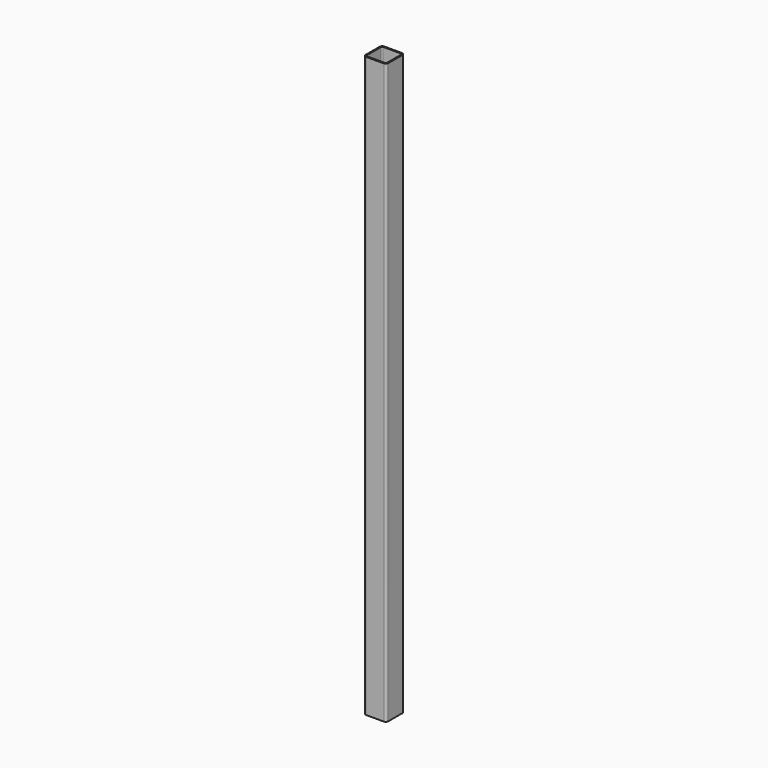
from build123d import *

# Parameters (mm, degrees)
F2_DEPTH = 812.8


# Not quite as in the source:
# - a variable given as a bare number and used for a length is read in inches; the dataset says mm whatever the document's units were


with BuildPart() as f2:
    # F0 (on Top) → F2 (new body)
    with BuildSketch(Plane.XY):
        with BuildLine():
            Line((-12.573, -15.875), (12.573, -15.875))
            ThreePointArc((12.573, -15.875), (14.9078665915, -14.9078665915), (15.875, -12.573))
            Line((15.875, -12.573), (15.875, 12.573))
            ThreePointArc((15.875, 12.573), (14.9078665915, 14.9078665915), (12.573, 15.875))
            Line((12.573, 15.875), (-12.573, 15.875))
            ThreePointArc((-12.573, 15.875), (-14.9078665915, 14.9078665915), (-15.875, 12.573))
            Line((-15.875, 12.573), (-15.875, -12.573))
            ThreePointArc((-15.875, -12.573), (-14.9078665915, -14.9078665915), (-12.573, -15.875))
        make_face()
        with BuildLine():
            Line((-12.573, 14.224), (12.573, 14.224))
            ThreePointArc((12.573, 14.224), (13.7404332957, 13.7404332957), (14.224, 12.573))
            Line((14.224, 12.573), (14.224, -12.573))
            ThreePointArc((14.224, -12.573), (13.7404332957, -13.7404332957), (12.573, -14.224))
            Line((12.573, -14.224), (-12.573, -14.224))
            ThreePointArc((-12.573, -14.224), (-13.7404332957, -13.7404332957), (-14.224, -12.573))
            Line((-14.224, -12.573), (-14.224, 12.573))
            ThreePointArc((-14.224, 12.573), (-13.7404332957, 13.7404332957), (-12.573, 14.224))
        make_face(mode=Mode.SUBTRACT)
    extrude(amount=F2_DEPTH)


solid = f2.part
